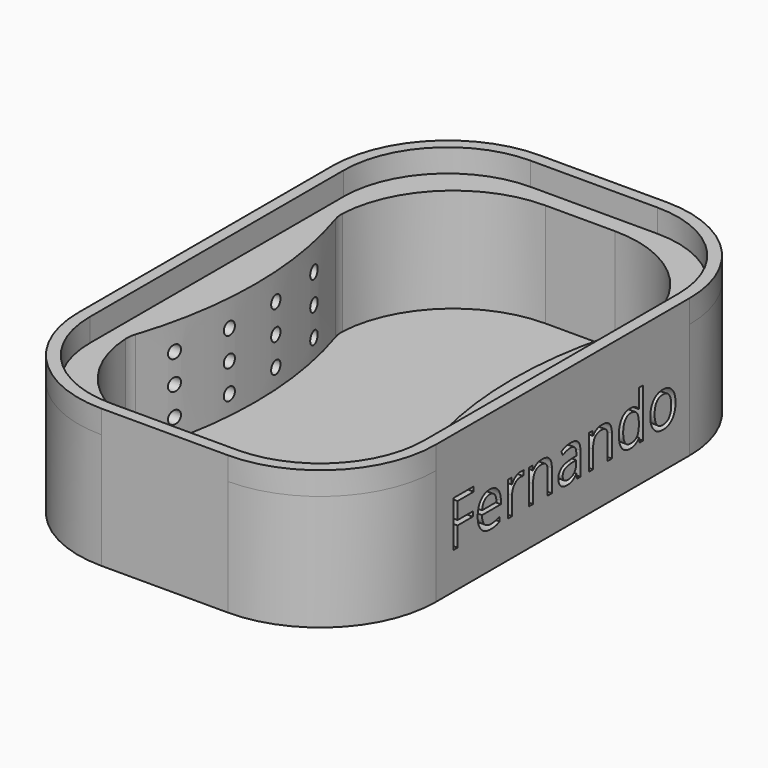
from build123d import *

# Parameters (mm, degrees)
F2_W         = 61.9495733385
F2_H         = 95
F3_DEPTH     = 20
F4_R         = 20
F5_DEPTH     = 18
F6_TEXT_SIZE = 11.1111111111
F7_DEPTH     = 18
F8_R         = 1.1037278567
F9_DEPTH     = 8.6016942646
F11_DEPTH    = 4


# Not quite as in the source:
# - Text() gives the source's letters only with a copy of the font that has no kerning and outlines rounded to 1/6400 em; it was checked with that copy


with BuildPart() as f3:
    # F2 (on offset) → F3 (new body)
    with BuildSketch(Plane.XY.offset(-20)):
        with Locations((26, 42.5)):
            Rectangle(F2_W, F2_H)
    extrude(amount=F3_DEPTH)

    # F4
    f4_edges = [f3.edges().sort_by_distance(p)[0] for p in [
        (-4.974787, 90, -10),
        (-4.974787, -5, -10),
        (56.974787, -5, -10),
        (56.974787, 90, -10),
    ]]
    fillet(f4_edges, radius=F4_R)

    # F1 (on Top) → F5 (cut)
    with BuildSketch(Plane.XY):
        with BuildLine():
            ThreePointArc((0.0252133308, 18.9960590063), (6.2173808707, 5.5072635456), (20, 0))
            Line((20, 0), (32, 0))
            ThreePointArc((32, 0), (45.7826191293, 5.5072635456), (51.9747866692, 18.9960590063))
            ThreePointArc((51.9747866692, 18.9960590063), (51.9372581584, 19.9076479214), (51.7347085296, 20.7972413044))
            ThreePointArc((51.7347085296, 20.7972413044), (48.2853679178, 42.5), (51.7347085296, 64.2027586956))
            ThreePointArc((51.7347085296, 64.2027586956), (51.9372581584, 65.0923520786), (51.9747866692, 66.0039409937))
            ThreePointArc((51.9747866692, 66.0039409937), (45.7826191293, 79.4927364544), (32, 85))
            Line((32, 85), (20, 85))
            ThreePointArc((20, 85), (6.2173808707, 79.4927364544), (0.0252133308, 66.0039409937))
            ThreePointArc((0.0252133308, 66.0039409937), (0.0627418416, 65.0923520786), (0.2652914704, 64.2027586956))
            ThreePointArc((0.2652914704, 64.2027586956), (3.7146320822, 42.5), (0.2652914704, 20.7972413044))
            ThreePointArc((0.2652914704, 20.7972413044), (0.0627418416, 19.9076479214), (0.0252133308, 18.9960590063))
        make_face()
    extrude(amount=-F5_DEPTH, mode=Mode.SUBTRACT)

    # F6 (on face) → F7 (cut)
    with BuildSketch(Plane.YZ.offset(56.9747866692)):
        with Locations((17.7070846967, -13.6365581653)):
            Text('Fernando', F6_TEXT_SIZE, font='Open Sans', text_align=(TextAlign.LEFT, TextAlign.BOTTOM))
    extrude(amount=-F7_DEPTH, mode=Mode.SUBTRACT)

    # F8 (on face) → F9 (cut, through all)
    with BuildSketch(Plane(origin=(-4.9747866692, 0, 0), x_dir=(0, -1, 0), z_dir=(-1, 0, 0))):
        with Locations((-57.1270175278, -14.627016373)):
            Circle(F8_R)
        with Locations((-57.1270175278, -9.627016373)):
            Circle(F8_R)
        with Locations((-57.1270175278, -4.627016373)):
            Circle(F8_R)
        with Locations((-47.1270175278, -14.627016373)):
            Circle(F8_R)
        with Locations((-47.1270175278, -9.627016373)):
            Circle(F8_R)
        with Locations((-47.1270175278, -4.627016373)):
            Circle(F8_R)
        with Locations((-37.1270175278, -14.627016373)):
            Circle(F8_R)
        with Locations((-37.1270175278, -9.627016373)):
            Circle(F8_R)
        with Locations((-37.1270175278, -4.627016373)):
            Circle(F8_R)
        with Locations((-27.1270175278, -14.627016373)):
            Circle(F8_R)
        with Locations((-27.1270175278, -9.627016373)):
            Circle(F8_R)
        with Locations((-27.1270175278, -4.627016373)):
            Circle(F8_R)
    extrude(amount=-F9_DEPTH, mode=Mode.SUBTRACT)

    # F10 (on face) → F11 (join)
    with BuildSketch(Plane.XY):
        with BuildLine():
            ThreePointArc((56.9747866692, 70), (51.116922293, 84.1421356237), (36.9747866692, 90))
            Line((36.9747866692, 90), (15.0252133308, 90))
            ThreePointArc((15.0252133308, 90), (0.883077707, 84.1421356237), (-4.9747866692, 70))
            Line((-4.9747866692, 70), (-4.9747866692, 15))
            ThreePointArc((-4.9747866692, 15), (0.883077707, 0.8578643763), (15.0252133308, -5))
            Line((15.0252133308, -5), (36.9747866692, -5))
            ThreePointArc((36.9747866692, -5), (51.116922293, 0.8578643763), (56.9747866692, 15))
            Line((56.9747866692, 15), (56.9747866692, 70))
        make_face()
        with BuildLine():
            ThreePointArc((-2.9747866692, 70), (2.2972912694, 82.7279220614), (15.0252133308, 88))
            Line((15.0252133308, 88), (36.9747866692, 88))
            ThreePointArc((36.9747866692, 88), (49.7027087306, 82.7279220614), (54.9747866692, 70))
            Line((54.9747866692, 70), (54.9747866692, 15))
            ThreePointArc((54.9747866692, 15), (49.7027087306, 2.2720779386), (36.9747866692, -3))
            Line((36.9747866692, -3), (15.0252133308, -3))
            ThreePointArc((15.0252133308, -3), (2.2972912694, 2.2720779386), (-2.9747866692, 15))
            Line((-2.9747866692, 15), (-2.9747866692, 70))
        make_face(mode=Mode.SUBTRACT)
    extrude(amount=F11_DEPTH)


solid = f3.part
